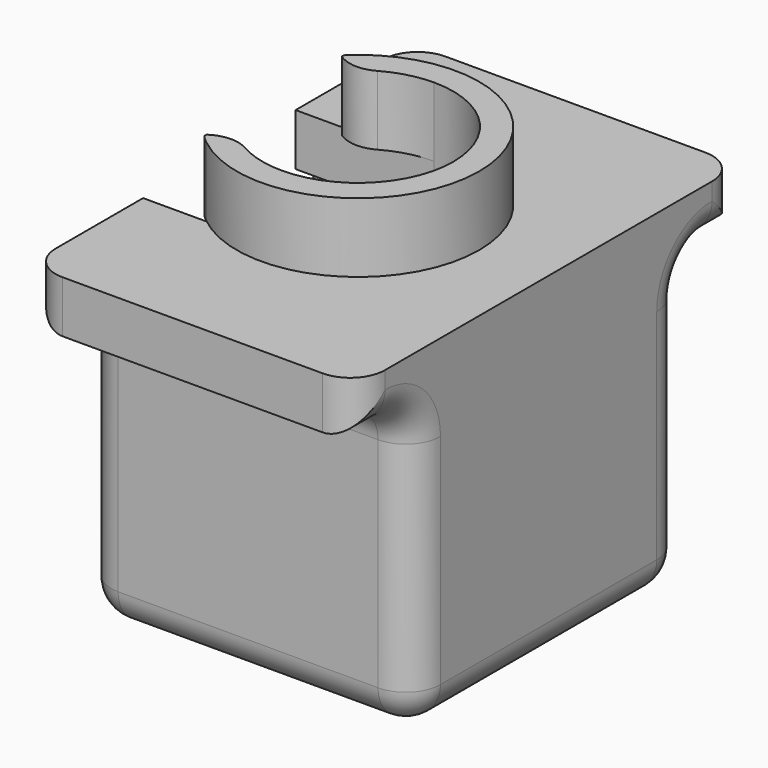
from build123d import *

# Parameters (mm, degrees)
F0_W      = 8
F0_H      = 6.8
F1_DEPTH  = 1.5
F2_DEPTH  = 6.8
F4_DEPTH  = 1.5
F6_DEPTH  = 2
F7_W      = 9.5
F7_H      = 1.5
F8_DEPTH  = 2
F9_W      = 9.5
F9_H      = 1.5
F10_DEPTH = 2
F11_F1_R  = 1
F11_F2_R  = 1


with BuildPart() as f1:
    # F0 (on Top) → F1 (new body)
    with BuildSketch(Plane.XY):
        Polygon((4, 3.4), (4, -3.4), (-4, -3.4), (-4, -4.9), (5.5, -4.9), (5.5, 4.9), (-4, 4.9), (-4, 3.4), align=None)
        Rectangle(F0_W, F0_H)
    extrude(amount=-F1_DEPTH)

    # F0 (on Top) → F2 (join)
    with BuildSketch(Plane.XY):
        Polygon((4, 3.4), (4, -3.4), (-4, -3.4), (-4, -4.9), (5.5, -4.9), (5.5, 4.9), (-4, 4.9), (-4, 3.4), align=None)
    extrude(amount=F2_DEPTH)

    # F3 (on face) → F4 (join)
    with BuildSketch(Plane.XY.offset(6.8)):
        with BuildLine():
            ThreePointArc((0, 2.75), (2.75, 0), (0, -2.75))
            Line((0, -2.75), (-4, -2.75))
            Line((-4, -2.75), (-4, -3.4))
            Line((-4, -3.4), (4, -3.4))
            Line((4, -3.4), (4, 3.4))
            Line((4, 3.4), (-4, 3.4))
            Line((-4, 3.4), (-4, 2.75))
            Line((-4, 2.75), (0, 2.75))
        make_face()
        Polygon((4, -3.4), (-4, -3.4), (-4, -4.9), (5.5, -4.9), (5.5, 4.9), (-4, 4.9), (-4, 3.4), (4, 3.4), align=None)
    extrude(amount=F4_DEPTH)

    # F5 (on face) → F6 (join)
    with BuildSketch(Plane.XY.offset(8.3)):
        with BuildLine():
            ThreePointArc((0, 2.75), (2.75, 0), (0, -2.75))
            Line((0, -2.75), (-2.1650635095, -2.75))
            ThreePointArc((-2.1650635095, -2.75), (3.5, 0), (-2.1650635095, 2.75))
            Line((-2.1650635095, 2.75), (0, 2.75))
        make_face()
        with BuildLine():
            ThreePointArc((-1.3555844547, 2.3926744004), (-0.7009441486, 2.6591685356), (0, 2.75))
            Line((0, 2.75), (-2.1650635095, 2.75))
            ThreePointArc((-2.1650635095, 2.75), (-2.2741617405, 2.6604864928), (-2.3795628172, 2.5666477747))
            ThreePointArc((-2.3795628172, 2.5666477747), (-2.4155229026, 2.507985001), (-2.4157537689, 2.4391780576))
            ThreePointArc((-2.4157537689, 2.4391780576), (-1.8923464861, 2.2636984741), (-1.3555844547, 2.3926744004))
        make_face()
        with BuildLine():
            ThreePointArc((0, -2.75), (-0.7009441486, -2.6591685356), (-1.3555844547, -2.3926744004))
            ThreePointArc((-1.3555844547, -2.3926744004), (-1.8923464861, -2.2636984741), (-2.4157537689, -2.4391780576))
            ThreePointArc((-2.4157537689, -2.4391780576), (-2.4155229026, -2.507985001), (-2.3795628172, -2.5666477747))
            ThreePointArc((-2.3795628172, -2.5666477747), (-2.2741617405, -2.6604864928), (-2.1650635095, -2.75))
            Line((-2.1650635095, -2.75), (0, -2.75))
        make_face()
    extrude(amount=F6_DEPTH)

    # F7 (on face) → F8 (join)
    with BuildSketch(Plane(origin=(0, 4.9, 0), x_dir=(-1, 0, 0), z_dir=(0, 1, 0))):
        with Locations((-0.75, 7.55)):
            Rectangle(F7_W, F7_H)
    extrude(amount=F8_DEPTH)

    # F9 (on face) → F10 (join)
    with BuildSketch(Plane.XZ.offset(4.9)):
        with Locations((0.75, 7.55)):
            Rectangle(F9_W, F9_H)
    extrude(amount=F10_DEPTH)

    # F11: fillet of radius 1 on 16 edges, made by hand

    # F11_f1
    f11_f1_edges = [f1.edges().sort_by_distance(p)[0] for p in [
        (0.75, -4.9, 6.8),
        (0.75, 4.9, 6.8),
    ]]
    fillet(f11_f1_edges, radius=F11_F1_R)

    # F11_f2
    f11_f2_edges = [f1.edges().sort_by_distance(p)[0] for p in [
        (0.75, -4.9, -1.5),
        (5.5, -4.9, 2.15),
        (5.5, 4.9, 2.15),
        (5.5, 0, -1.5),
        (0.75, 4.9, -1.5),
        (-4, 4.9, 2.15),
        (-4, 0, -1.5),
        (-4, -4.9, 2.15),
        (-4, 6.9, 7.55),
        (-4, 6.4, 6.8),
        (5.5, 6.9, 7.55),
        (5.5, -6.9, 7.55),
        (-4, -6.9, 7.55),
        (-4, -6.4, 6.8),
        (-4, -5.1928932188, 6.5071067812),
        (-4, 5.1928932188, 6.5071067812),
        (5.5, 5.1928932188, 6.5071067812),
        (5.5, -5.1928932188, 6.5071067812),
    ]]
    fillet(f11_f2_edges, radius=F11_F2_R)


solid = f1.part
